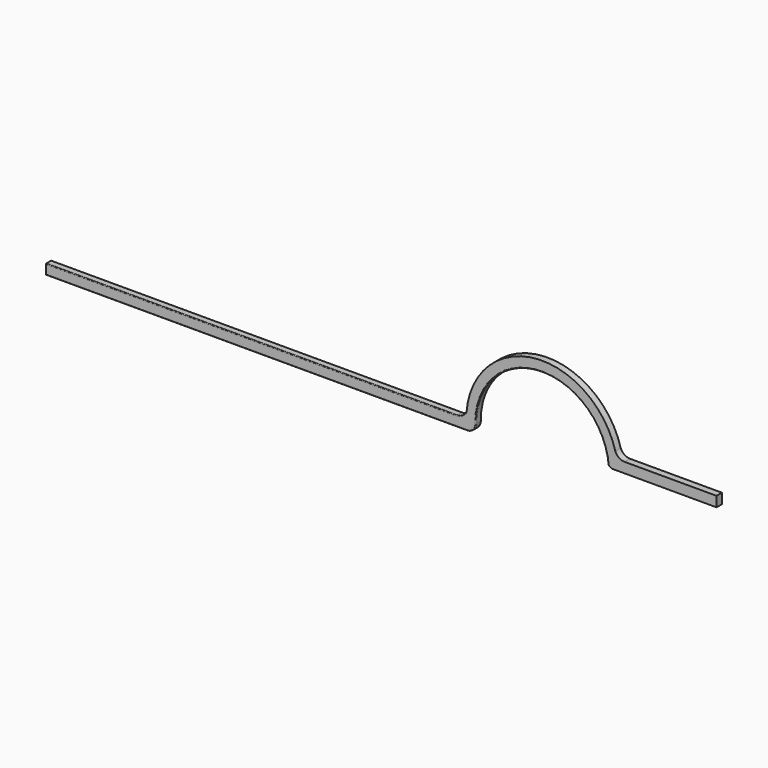
from build123d import *

# Parameters (mm, degrees)
F1_DEPTH = 50.8
F2_T     = -6.35
F3_R     = 5.08


# Not quite as in the source:
# - a feature names something its author has since deleted; it is built from what else it names


with BuildPart() as f1:
    # F0 (on Front) → F1 (new body)
    with BuildSketch(Plane.XZ):
        with BuildLine():
            Line((-2514.6, 38.1), (-2514.6, -38.1))
            Line((-2514.6, -38.1), (642.62, -38.1))
            ThreePointArc((642.62, -38.1), (689.5262652886, -18.5474593485), (708.6573440579, 28.5322750855))
            ThreePointArc((708.6573440579, 28.5322750855), (1175.5106386372, 529.8946007496), (1701.0397320407, 90.4229267577))
            ThreePointArc((1701.0397320407, 90.4229267577), (1714.8164995695, 70.9613276191), (1737.4633923968, 63.5))
            Line((1737.4633923968, 63.5), (2514.6, 63.5))
            Line((2514.6, 63.5), (2514.6, 139.7))
            Line((2514.6, 139.7), (1826.26, 139.7))
            ThreePointArc((1826.26, 139.7), (1783.3875941693, 152.9047873384), (1755.3740072802, 187.9426031947))
            ThreePointArc((1755.3740072802, 187.9426031947), (1160.1113564946, 605.1657592852), (640.5706087962, 96.7464472213))
            ThreePointArc((640.5706087962, 96.7464472213), (613.6897539567, 54.5337021318), (566.42, 38.1))
            Line((566.42, 38.1), (-2514.6, 38.1))
        make_face()
    extrude(amount=F1_DEPTH)

    # F2
    f2_openings = [f1.faces().sort_by_distance(p)[0] for p in [
        (-2514.6, -25.4, 0),
    ]]
    offset(amount=F2_T, openings=f2_openings, kind=Kind.INTERSECTION)

    # F3
    f3_edges = [f1.edges().sort_by_distance(p)[0] for p in [
        (-974.09, -50.8, 38.1),
        (-974.09, 0, 38.1),
        (-935.99, 0, -38.1),
        (-935.99, -50.8, -38.1),
    ]]
    fillet(f3_edges, radius=F3_R)


solid = f1.part
